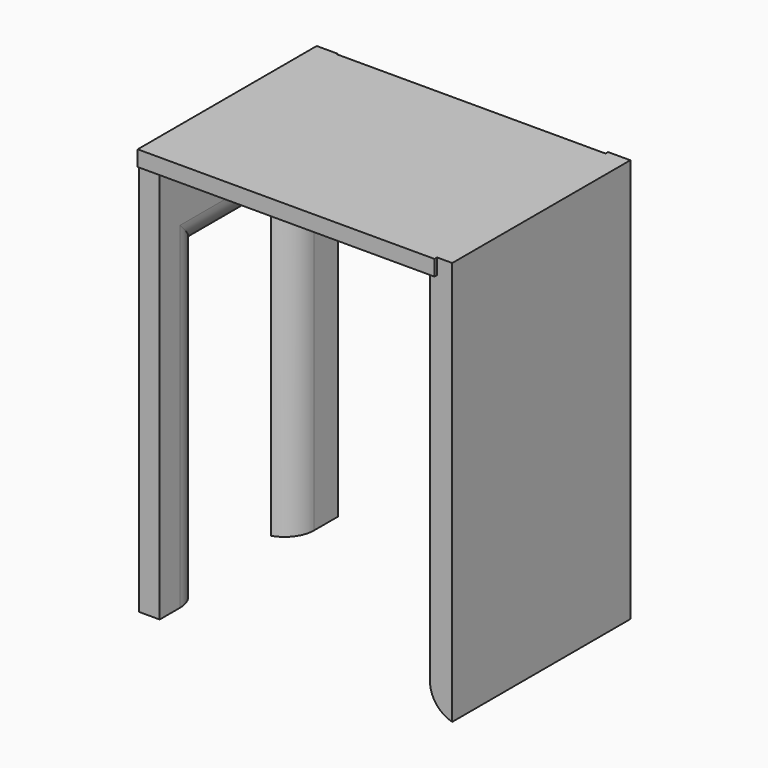
from build123d import *

# Parameters (mm, degrees)
F0_W           = 50.8
F0_H           = 38.1
F1_DEPTH       = 3.175
F3_START       = -18.288
F2_W           = 38.1
F2_H           = 69.85
F3_DEPTH       = 3.556
F5_START       = 27.686
F4_W           = 38.1
F4_H           = 69.85
F5_DEPTH       = 3.81
F6_W           = 19.05
F6_H           = 53.975
F7_DEPTH       = 32.004
F8_T1_DEPTH    = 64.9044340938
F8_T3_DEPTH    = 19.05
F8_T5_DEPTH    = 62.6934442484
F8_T11_DEPTH   = 64.9044340938
F8_T15_DEPTH   = 31.165027858
F8_T23_DEPTH   = 31.165027858
F8_T28_DEPTH   = 64.9044340938
F9_W           = 54.9304988235
F9_H           = 1.4888443984
F10_DEPTH      = 28.4988
F10_DEPTH_BACK = 25.4


# Not quite as in the source:
# - a fillet or chamfer that OpenCascade refuses, or shapes differently, is made with other operations: its cross-section is extruded or revolved along the edge and cut away or added


with BuildPart() as f1:
    # F0 (on Top) → F1 (new body)
    with BuildSketch(Plane.XY):
        with Locations((3.5055922344, 6.6658267866)):
            Rectangle(F0_W, F0_H)
    extrude(amount=F1_DEPTH)

    # F2 (on Right) → F3 (join)
    with BuildSketch(Plane.YZ.offset(F3_START)):
        with Locations((6.8596902806, -32.1689685807)):
            Rectangle(F2_W, F2_H)
    extrude(amount=-F3_DEPTH)

    # F4 (on Right) → F5 (join)
    with BuildSketch(Plane.YZ.offset(F5_START)):
        with Locations((7.2173965164, -31.5503366292)):
            Rectangle(F4_W, F4_H)
    extrude(amount=F5_DEPTH)

    # F6 (on Right) → F7 (cut)
    with BuildSketch(Plane.YZ):
        with Locations((6.4956571441, -41.2920623448)):
            Rectangle(F6_W, F6_H)
    extrude(amount=-F7_DEPTH, mode=Mode.SUBTRACT)

    # F8: fillet of radius 5.08 on 4 edges, made by hand

    # F8_s2 → F8_t1 (cut)
    with BuildSketch(Plane.XY.offset(-79.2089964387)):
        with BuildLine():
            ThreePointArc((-18.288, 20.8666682873), (-19.2723730639, 17.8612997575), (-21.844, 16.0206571441))
            Line((-21.844, 16.0206571441), (-18.288, 16.0206571441))
            Line((-18.288, 16.0206571441), (-18.288, 20.8666682873))
        make_face()
        with BuildLine():
            ThreePointArc((-18.288, -7.8753539991), (-19.2723730639, -4.8699854693), (-21.844, -3.0293428559))
            Line((-21.844, -3.0293428559), (-18.288, -3.0293428559))
            Line((-18.288, -3.0293428559), (-18.288, -7.8753539991))
        make_face()
    extrude(amount=F8_T1_DEPTH, mode=Mode.SUBTRACT)

    # F8_s4 → F8_t3 (cut)
    with BuildSketch(Plane.XZ.offset(-16.0206571441)):
        with BuildLine():
            ThreePointArc((-18.288, -9.4585512016), (-19.2723730639, -12.4639197314), (-21.844, -14.3045623448))
            Line((-21.844, -14.3045623448), (-18.288, -14.3045623448))
            Line((-18.288, -14.3045623448), (-18.288, -9.4585512016))
        make_face()
    extrude(amount=F8_T3_DEPTH, mode=Mode.SUBTRACT)

    # F8_s6 → F8_t5 (cut)
    with BuildSketch(Plane.XZ.offset(-38.5641186406)):
        with BuildLine():
            ThreePointArc((27.686, -61.5566477795), (28.7499073716, -64.6674997528), (31.496, -66.4753366292))
            Line((31.496, -66.4753366292), (27.686, -66.4753366292))
            Line((27.686, -66.4753366292), (27.686, -61.5566477795))
        make_face()
    extrude(amount=F8_T5_DEPTH, mode=Mode.SUBTRACT)


with BuildPart() as f8_tool9:
    # F8_s10 → F8_t11 (new body)
    with BuildSketch(Plane.XY.offset(-67.0939685807)):
        with BuildLine():
            ThreePointArc((-18.288, 20.8666682873), (-19.2723730639, 17.8612997575), (-21.844, 16.0206571441))
            Line((-21.844, 16.0206571441), (-18.288, 16.0206571441))
            Line((-18.288, 16.0206571441), (-18.288, 20.8666682873))
        make_face()
    extrude(amount=F8_T11_DEPTH)

    split(bisect_by=Plane.XY.offset(-14.3045623448), keep=Keep.TOP)


with BuildPart() as f8_tool13:
    # F8_s14 → F8_t15 (new body)
    with BuildSketch(Plane.XZ.offset(-28.1356850021)):
        with BuildLine():
            ThreePointArc((-18.288, -9.4585512016), (-19.2723730639, -12.4639197314), (-21.844, -14.3045623448))
            Line((-21.844, -14.3045623448), (-18.288, -14.3045623448))
            Line((-18.288, -14.3045623448), (-18.288, -9.4585512016))
        make_face()
    extrude(amount=F8_T15_DEPTH)

    split(bisect_by=Plane.XZ.offset(-25.9096902806), keep=Keep.TOP)

    split(bisect_by=Plane.XZ.offset(-16.0206571441), keep=Keep.BOTTOM)


with BuildPart() as f8_tool9_1:
    add(f8_tool9.part)

    # F8_t18: intersect F8_tool13
    add(f8_tool13.part, mode=Mode.INTERSECT)


with BuildPart() as f1_1:
    add(f1.part)

    # F8_t7: cut F8_tool9
    add(f8_tool9_1.part, mode=Mode.SUBTRACT)


with BuildPart() as f8_tool21:
    # F8_s22 → F8_t23 (new body)
    with BuildSketch(Plane.XZ.offset(-16.0206571441)):
        with BuildLine():
            ThreePointArc((-18.288, -9.4585512016), (-19.2723730639, -12.4639197314), (-21.844, -14.3045623448))
            Line((-21.844, -14.3045623448), (-18.288, -14.3045623448))
            Line((-18.288, -14.3045623448), (-18.288, -9.4585512016))
        make_face()
    extrude(amount=F8_T23_DEPTH)

    split(bisect_by=Plane.XZ.offset(12.1903097194), keep=Keep.BOTTOM)

    split(bisect_by=Plane.XZ.offset(3.0293428559), keep=Keep.TOP)


with BuildPart() as f8_tool26:
    # F8_s27 → F8_t28 (new body)
    with BuildSketch(Plane.XY.offset(-2.1895344868)):
        with BuildLine():
            ThreePointArc((-18.288, -7.8753539991), (-19.2723730639, -4.8699854693), (-21.844, -3.0293428559))
            Line((-21.844, -3.0293428559), (-18.288, -3.0293428559))
            Line((-18.288, -3.0293428559), (-18.288, -7.8753539991))
        make_face()
    extrude(amount=-F8_T28_DEPTH)

    split(bisect_by=Plane.XY.offset(-14.3045623448), keep=Keep.TOP)


with BuildPart() as f8_tool21_1:
    add(f8_tool21.part)

    # F8_t30: intersect F8_tool26
    add(f8_tool26.part, mode=Mode.INTERSECT)


with BuildPart() as f1_2:
    add(f1_1.part)

    # F8_t19: cut F8_tool21
    add(f8_tool21_1.part, mode=Mode.SUBTRACT)

    # F9 (on Front) → F10 (cut, two sides)
    with BuildSketch(Plane.XZ) as f10_sk:
        with Locations((4.6410532668, 3.4134599846)):
            Rectangle(F9_W, F9_H)
    extrude(amount=-F10_DEPTH, mode=Mode.SUBTRACT)
    extrude(f10_sk.sketch, amount=F10_DEPTH_BACK, mode=Mode.SUBTRACT)


solid = f1_2.part
